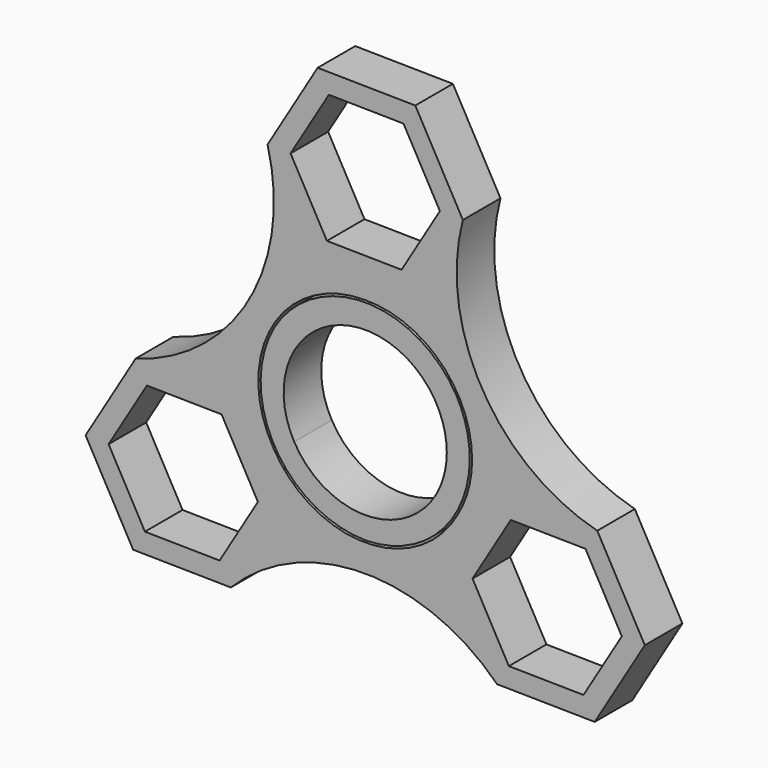
from build123d import *

# Parameters (mm, degrees)
F1_DEPTH = 6.35


# Not quite as in the source:
# - a feature names something its author has since deleted; it is built from what else it names


with BuildPart() as f1:
    # F0 (on Front) → F1 (new body)
    with BuildSketch(Plane.XZ):
        with BuildLine():
            ThreePointArc((14.1278163557, 0.2731498923), (13.651376792, 3.9320111734), (12.2538333812, 7.346851279))
            ThreePointArc((12.2538333812, 7.346851279), (-0.0774496188, 14.2872900792), (-12.3327636124, 7.2135704011))
            ThreePointArc((-12.3327636124, 7.2135704011), (-12.1777184268, -6.9358533383), (0.0759595105, -14.012406749))
            ThreePointArc((0.0759595105, -14.012406749), (10.026076215, -9.745979428), (14.1278163557, 0.2731498923))
        make_face()
        with BuildLine():
            ThreePointArc((11.1803129237, 0.2748650387), (10.7918465004, -2.6257712301), (9.6538259749, -5.3219734128))
            ThreePointArc((9.6538259749, -5.3219734128), (0.0597566836, -11.0234380344), (-9.5955608055, -5.4263219393))
            ThreePointArc((-9.5955608055, -5.4263219393), (-9.736139361, 5.7331181035), (-0.0612358901, 11.2963102831))
            ThreePointArc((-0.0612358901, 11.2963102831), (7.874134009, 8.1464067398), (11.1803129237, 0.2748650387))
        make_face(mode=Mode.SUBTRACT)
        with BuildLine():
            ThreePointArc((9.4358771612, 5.6994718316), (10.6192535621, 2.9582445374), (11.0236, 0))
            ThreePointArc((11.0236, 0), (10.6756656227, -2.7477118611), (9.6538259749, -5.3219734128))
            ThreePointArc((9.6538259749, -5.3219734128), (10.7918465004, -2.6257712301), (11.1803129237, 0.2748650387))
            ThreePointArc((11.1803129237, 0.2748650387), (7.874134009, 8.1464067398), (-0.0612358901, 11.2963102831))
            ThreePointArc((-0.0612358901, 11.2963102831), (5.4371548072, 9.7702629436), (9.4358771612, 5.6994718316))
        make_face()
        with BuildLine():
            ThreePointArc((-9.4971130513, 5.5968384515), (-0.0597566836, 11.0234380344), (9.4358771612, 5.6994718316))
            ThreePointArc((9.4358771612, 5.6994718316), (5.4371548072, 9.7702629436), (-0.0612358901, 11.2963102831))
            ThreePointArc((-0.0612358901, 11.2963102831), (-5.542758908, 9.7107421999), (-9.4971130513, 5.5968384515))
        make_face()
        with BuildLine():
            ThreePointArc((-9.5955608055, -5.4263219393), (-11.0231603907, 0.0984477542), (-9.4971130513, 5.5968384515))
            ThreePointArc((-9.4971130513, 5.5968384515), (-5.542758908, 9.7107421999), (-0.0612358901, 11.2963102831))
            ThreePointArc((-0.0612358901, 11.2963102831), (-9.736139361, 5.7331181035), (-9.5955608055, -5.4263219393))
        make_face()
    extrude(amount=F1_DEPTH)


with BuildPart() as f1b:
    # F0 (on Front) → F1, piece 2 (new body)
    with BuildSketch(Plane.XZ):
        with BuildLine():
            ThreePointArc((31.3557710331, -2.6839999789), (15.827926935, 9.0774163735), (13.1967604274, 28.378240702))
            Line((13.1967604274, 28.378240702), (6.4279816632, 17.0478905732))
            Line((6.4279816632, 17.0478905732), (-6.7687787642, 17.2446498712))
            Line((-6.7687787642, 17.2446498712), (-13.1967604274, 28.771759298))
            ThreePointArc((-13.1967604274, 28.771759298), (-15.7087414623, 9.494980858), (-31.0179446527, -2.4855255345))
            Line((-31.0179446527, -2.4855255345), (-17.8211842253, -2.6822848325))
            Line((-17.8211842253, -2.6822848325), (-11.3932025621, -14.2093942593))
            Line((-11.3932025621, -14.2093942593), (-18.1619813263, -25.5397443881))
            ThreePointArc((-18.1619813263, -25.5397443881), (-0.2123739316, -17.9729451093), (17.8182135046, -25.3447002365))
            Line((17.8182135046, -25.3447002365), (11.3902318414, -13.8175908097))
            Line((11.3902318414, -13.8175908097), (18.1590106056, -2.4872406809))
            Line((18.1590106056, -2.4872406809), (31.3557710331, -2.6839999789))
        make_face()
        with BuildLine():
            ThreePointArc((14.4442129237, 0.2748650387), (13.9468727552, -3.4619983612), (12.489476536, -6.9387053624))
            ThreePointArc((12.489476536, -6.9387053624), (0.0774496188, -14.2872900792), (-12.4135170255, -7.0737013866))
            ThreePointArc((-12.4135170255, -7.0737013866), (-12.5715646135, 7.3497215946), (-0.0789302311, 14.5604216801))
            ThreePointArc((-0.0789302311, 14.5604216801), (10.175842244, 10.460624898), (14.4442129237, 0.2748650387))
        make_face(mode=Mode.SUBTRACT)
        Polygon((6.4279816632, 17.0478905732), (13.1967604274, 28.378240702), (6.7687787642, 39.9053501288), (-6.4279816632, 40.1021094268), (-13.1967604274, 28.771759298), (-6.7687787642, 17.2446498712), align=None)
        Polygon((5.1762630455, 37.2352832458), (10.0881568176, 28.4223663289), (4.9118937721, 19.7620830831), (-5.1762630455, 19.9147167542), (-10.0881568176, 28.7276336711), (-4.9118937721, 37.3879169169), align=None, mode=Mode.SUBTRACT)
        Polygon((37.7837526963, -14.2111094057), (31.3557710331, -2.6839999789), (18.1590106056, -2.4872406809), (11.3902318414, -13.8175908097), (17.8182135046, -25.3447002365), (31.0149739321, -25.5414595345), align=None)
        Polygon((14.4988354513, -13.8617164365), (19.6750984967, -5.2014331907), (29.7632553143, -5.3540668619), (34.6751490864, -14.1669837788), (29.4988860409, -22.8272670246), (19.4107292234, -22.6746333535), align=None, mode=Mode.SUBTRACT)
        Polygon((-17.8211842253, -2.6822848325), (-31.0179446527, -2.4855255345), (-37.7867234169, -13.8158756633), (-31.3587417537, -25.3429850901), (-18.1619813263, -25.5397443881), (-11.3932025621, -14.2093942593), align=None)
        Polygon((-19.413699944, -5.3523517155), (-14.5018061719, -14.1652686324), (-19.6780692174, -22.8255518782), (-29.7662260349, -22.6729182071), (-34.678119807, -13.8600012902), (-29.5018567616, -5.1997180444), align=None, mode=Mode.SUBTRACT)
    extrude(amount=F1_DEPTH)


solid = Compound([f1.part, f1b.part])
